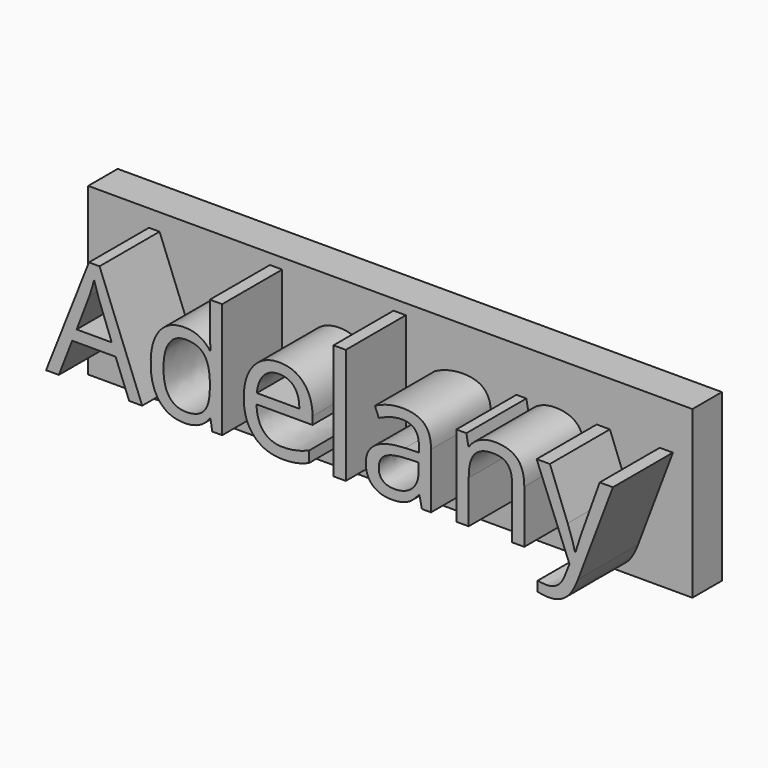
from build123d import *

# Parameters (mm, degrees)
F0_TEXT_SIZE = 51.413614872
F1_DEPTH     = 25.4
F2_W         = 204.5674175024
F2_H         = 56.2366936356
F3_DEPTH     = 12.48672


# Not quite as in the source:
# - Text() gives the source's letters only with a copy of the font that has no kerning and outlines rounded to 1/6400 em; it was checked with that copy


with BuildPart() as f1:
    # F0 (on Front) → F1 (new body)
    with BuildSketch(Plane.XZ):
        with Locations((-73.8013237715, 5.5058123544)):
            Text('Adelany', F0_TEXT_SIZE, font='Open Sans', text_align=(TextAlign.LEFT, TextAlign.BOTTOM))
    extrude(amount=F1_DEPTH)


with BuildPart() as f3:
    # F2 (on Front) → F3 (new body)
    with BuildSketch(Plane.XZ):
        with Locations((22.4188938737, 20.0319541618)):
            Rectangle(F2_W, F2_H)
    extrude(amount=-F3_DEPTH)


solid = Compound([f1.part, f3.part])
